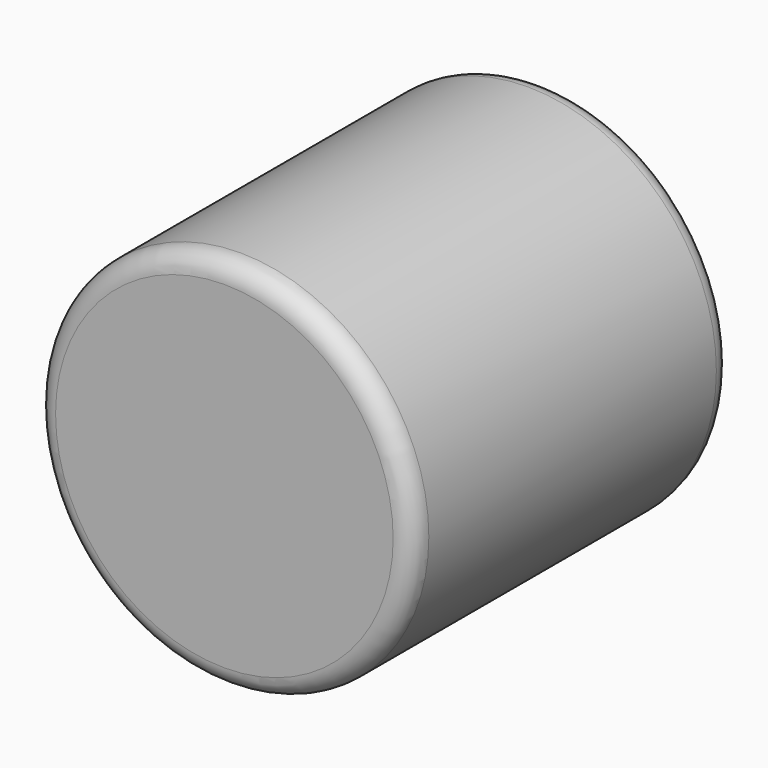
from build123d import *

# Parameters (mm, degrees)
F0_R     = 48.3453961675
F1_DEPTH = 50.8
F2_T     = -2.54


# Not quite as in the source:
# - a fillet or chamfer that OpenCascade refuses, or shapes differently, is made with other operations: its cross-section is extruded or revolved along the edge and cut away or added


with BuildPart() as f1:
    # F0 (on Front) → F1 (new body, symmetric)
    with BuildSketch(Plane.XZ):
        Circle(F0_R)
    extrude(amount=F1_DEPTH, both=True)

    # F2
    f2_openings = [f1.faces().sort_by_distance(p)[0] for p in [
        (0, 50.8, 0),
    ]]
    offset(amount=F2_T, openings=f2_openings)

    # F3: fillet of radius 5.08 on 3 edges, made by hand

    # F3_s1 → F3_t2 (revolve, cut)
    with BuildSketch(Plane.XY):
        with BuildLine():
            ThreePointArc((48.3453961675, 46.4005909488), (47.6648052188, 48.9405909488), (45.8053961675, 50.8))
            Line((45.8053961675, 50.8), (45.8561961675, 50.887988181))
            ThreePointArc((45.8561961675, 50.887988181), (47.0753961675, 50.9016), (48.3453961675, 50.9016))
            Line((48.3453961675, 50.9016), (48.4469961675, 50.8))
            Line((48.4469961675, 50.8), (48.4469961675, 46.4005909488))
            Line((48.4469961675, 46.4005909488), (48.3453961675, 46.4005909488))
        make_face()
    revolve(axis=Axis((0, 50.8, 0), (0, -1, 0)), mode=Mode.SUBTRACT)

    # F3_s3 → F3_t4 (revolve, cut)
    with BuildSketch(Plane.XY):
        with BuildLine():
            ThreePointArc((48.3453961675, -45.72), (46.857498616, -49.3121024484), (43.2653961675, -50.8))
            Line((43.2653961675, -50.8), (43.2653961675, -50.9016))
            Line((43.2653961675, -50.9016), (48.4469961675, -50.9016))
            Line((48.4469961675, -50.9016), (48.4469961675, -45.72))
            Line((48.4469961675, -45.72), (48.3453961675, -45.72))
        make_face()
    revolve(axis=Axis((0, -50.8, 0), (0, -1, 0)), mode=Mode.SUBTRACT)


solid = f1.part
